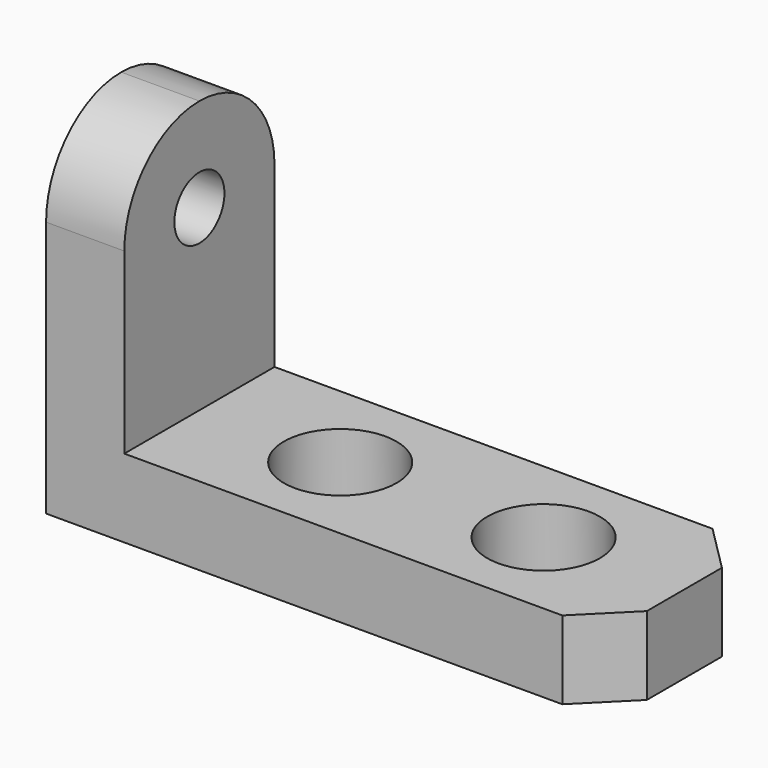
from build123d import *

# Parameters (mm, degrees)
F0_W     = 180
F0_H     = 60
F1_DEPTH = 25
F2_W     = 25
F2_H     = 60
F3_DEPTH = 87
F4_R     = 29.99999
F5_SIZE  = 15
F6_R     = 18
F7_DEPTH = 25
F8_R     = 10
F9_DEPTH = 25.001


# Not quite as in the source:
# - a fillet or chamfer is up to 0.001 mm smaller than in the source, because OpenCascade refuses the exact size


with BuildPart() as f1:
    # F0 (on Top) → F1 (new body)
    with BuildSketch(Plane.XY):
        with Locations((90, 30)):
            Rectangle(F0_W, F0_H)
    extrude(amount=F1_DEPTH)

    # F2 (on face) → F3 (join)
    with BuildSketch(Plane.XY.offset(25)):
        with Locations((12.5, 30)):
            Rectangle(F2_W, F2_H)
    extrude(amount=F3_DEPTH)

    # F4 (radius 30 in the source; OpenCascade refuses exactly that, so slightly less here)
    f4_edges = [f1.edges().sort_by_distance(p)[0] for p in [
        (12.5, 0, 112),
        (12.5, 60, 112),
    ]]
    fillet(f4_edges, radius=F4_R)

    # F5
    f5_edges = [f1.edges().sort_by_distance(p)[0] for p in [
        (180, 0, 12.5),
        (180, 60, 12.5),
    ]]
    chamfer(f5_edges, length=F5_SIZE)

    # F6 (on face) → F7 (cut)
    with BuildSketch(Plane.XY.offset(25)):
        with Locations((70, 30)):
            Circle(F6_R)
        with Locations((135, 30)):
            Circle(F6_R)
    extrude(amount=-F7_DEPTH, mode=Mode.SUBTRACT)

    # F8 (on face) → F9 (cut, through all)
    with BuildSketch(Plane.YZ.offset(25)):
        with Locations((30, 82)):
            Circle(F8_R)
    extrude(amount=-F9_DEPTH, mode=Mode.SUBTRACT)


solid = f1.part
